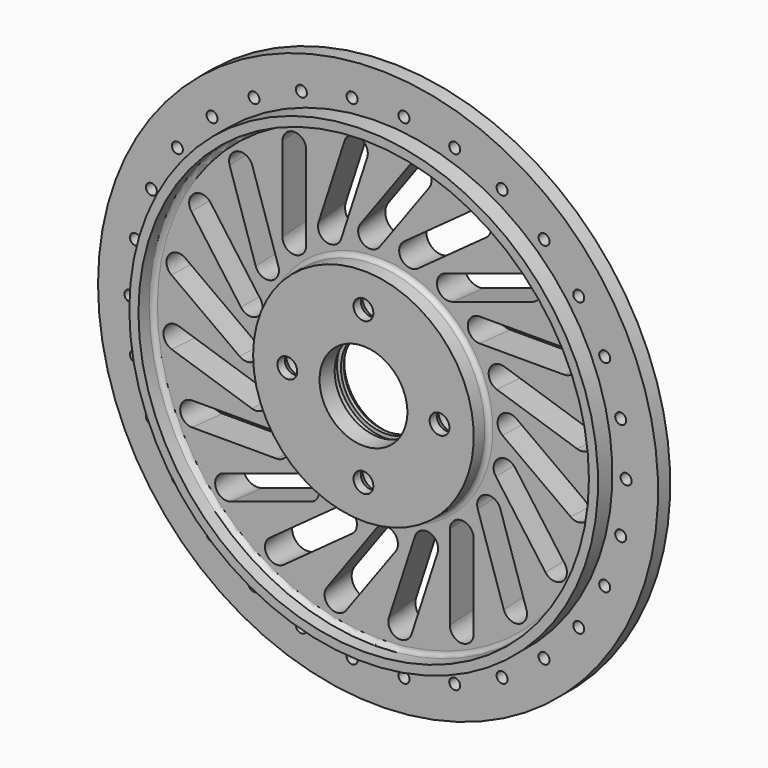
from build123d import *

# Parameters (mm, degrees)
F2_R            = 3.6
F3_DEPTH        = 50
F3_COPIES_COUNT = 30
F5_COPIES_COUNT = 4
F7_DEPTH        = 37.001
F7_TAPER        = 5
F7_COPIES_COUNT = 20


# Not quite as in the source:
# - a pattern or mirror of a feature is missing from the dataset's text; its kind, count and spacing are read off the source's solid


with BuildPart() as f1:
    # F0 (on Top) → F1 (revolve)
    with BuildSketch(Plane.XY):
        with BuildLine():
            ThreePointArc((-75.5, 12), (-73.3786796564, 11.1213203436), (-72.5, 9))
            Line((-72.5, 9), (-72.5, 0))
            Line((-72.5, 0), (-28.85, 0))
            Line((-28.85, 0), (-28.85, 12.4))
            Line((-28.85, 12.4), (-31.45, 12.4))
            Line((-31.45, 12.4), (-31.45, 17.6))
            Line((-31.45, 17.6), (-28.85, 17.6))
            Line((-28.85, 17.6), (-28.85, 20))
            Line((-28.85, 20), (-30, 20))
            ThreePointArc((-30, 20), (-30.7071067812, 20.2928932188), (-31, 21))
            Line((-31, 21), (-31, 23))
            Line((-31, 23), (-67.5, 37))
            Line((-67.5, 37), (-154, 37))
            Line((-154, 37), (-154, 22))
            Line((-154, 22), (-184, 22))
            Line((-184, 22), (-184, 12))
            Line((-184, 12), (-154, 12))
            Line((-154, 12), (-154, 0.2))
            Line((-154, 0.2), (-148, 0.2))
            Line((-148, 0.2), (-148, 9))
            ThreePointArc((-148, 9), (-147.1213203436, 11.1213203436), (-145, 12))
            Line((-145, 12), (-75.5, 12))
        make_face()
    revolve(axis=Axis((0, 8.013517431, 0), (0, -1, 0)))

    # F2 (on Front) → F3 (cut)
    with BuildSketch(Plane.XZ):
        with Locations((163, 0)):
            Circle(F2_R)
    f3 = extrude(amount=-F3_DEPTH, mode=Mode.SUBTRACT)

    # F3_copies: F3 ×30 about axis
    f3_copies_axis = Axis((0, 0, 0), (0, 1, 0))
    for i in range(1, F3_COPIES_COUNT):
        add(f3.rotate(f3_copies_axis, i * 360 / F3_COPIES_COUNT), mode=Mode.SUBTRACT)

    # F4 (on Right) → F5 (revolve, cut)
    with BuildSketch(Plane.YZ):
        Polygon((0, 56.5), (0, 50), (51.0571013514, 50), (51.0571013514, 59), (10.3301270189, 59), (6, 56.5), align=None)
    f5 = revolve(axis=Axis((0, 25.5285506757, 50), (0, 1, 0)), mode=Mode.SUBTRACT)

    # F5_copies: F5 ×4 about axis
    f5_copies_axis = Axis((0, 0, 0), (0, 1, 0))
    for i in range(1, F5_COPIES_COUNT):
        add(f5.rotate(f5_copies_axis, i * 360 / F5_COPIES_COUNT), mode=Mode.SUBTRACT)

    # F6 (on face) → F7 (cut, through all)
    with BuildSketch(Plane(origin=(0, 37, 0), x_dir=(-1, 0, 0), z_dir=(0, 1, 0))):
        with BuildLine():
            Line((65, 66.7626392528), (65, 122.1924711265))
            ThreePointArc((65, 122.1924711265), (55, 132.1924711265), (45, 122.1924711265))
            Line((45, 122.1924711265), (45, 66.7626392528))
            ThreePointArc((45, 66.7626392528), (55, 56.7626392528), (65, 66.7626392528))
        make_face()
    f7 = extrude(amount=-F7_DEPTH, taper=F7_TAPER, mode=Mode.SUBTRACT)

    # F7_copies: F7 ×20 about axis
    f7_copies_axis = Axis((0, 0, 0), (0, 1, 0))
    for i in range(1, F7_COPIES_COUNT):
        add(f7.rotate(f7_copies_axis, i * 360 / F7_COPIES_COUNT), mode=Mode.SUBTRACT)


solid = f1.part
